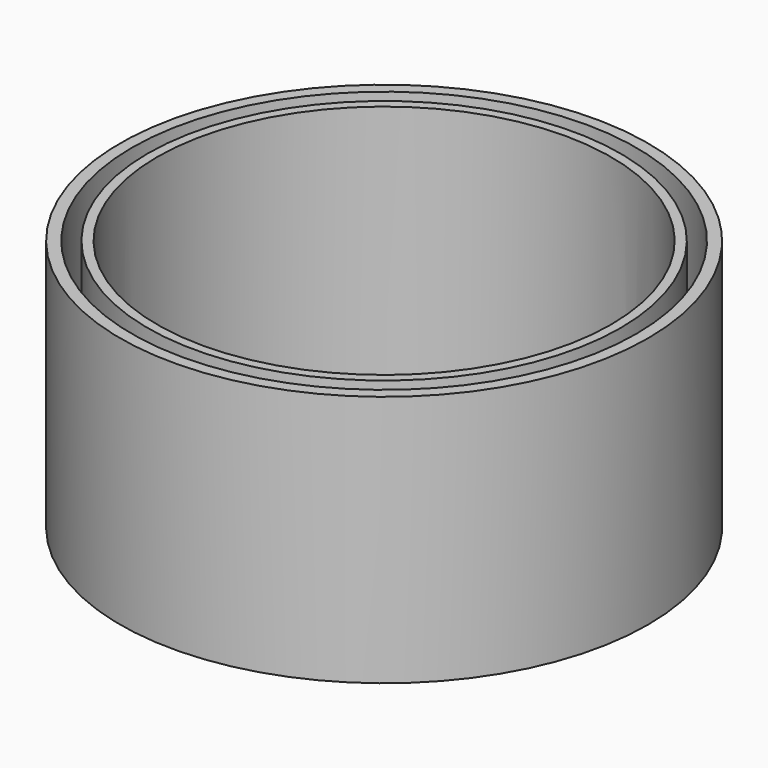
from build123d import *

# Parameters (mm, degrees)
F0_R      = 33.5
F0_R_2    = 32
F1_DEPTH  = 30
F0_R_3    = 30
F0_R_4    = 28.8
F2_R      = 33.5
F3_DEPTH  = 2
F5_DEPTH  = 12
F6_SIZE   = 11.9999
F6_2_SIZE = 11.9999
F6_3_SIZE = 11.9999
F8_R      = 6.5
F9_DEPTH  = 25


# Not quite as in the source:
# - a fillet or chamfer is up to 0.001 mm smaller than in the source, because OpenCascade refuses the exact size


with BuildPart() as f1:
    # F0 (on Top) → F1 (new body)
    with BuildSketch(Plane.XY):
        Circle(F0_R)
        Circle(F0_R_2, mode=Mode.SUBTRACT)
    extrude(amount=F1_DEPTH)


with BuildPart() as f1b:
    # F0 (on Top) → F1, piece 2 (new body)
    with BuildSketch(Plane.XY):
        Circle(F0_R_3)
        Circle(F0_R_4, mode=Mode.SUBTRACT)
    extrude(amount=F1_DEPTH)


with BuildPart() as f3:
    # F2 (on face) → F3 (new body)
    with BuildSketch(Plane(origin=(0, 0, 0), x_dir=(1, 0, 0), z_dir=(0, 0, -1))):
        Circle(F2_R)
    extrude(amount=F3_DEPTH)


with BuildPart() as f5:
    # F4 (on face) → F5 (new body)
    with BuildSketch(Plane.XY):
        with BuildLine():
            Line((9.993418715, 25.1754931604), (10.5667748746, 26.7914775395))
            ThreePointArc((10.5667748746, 26.7914775395), (10.0999818657, 26.9709170462), (9.630143492, 27.1422242332))
            Line((9.630143492, 27.1422242332), (9.993418715, 25.1754931604))
        make_face()
        with BuildLine():
            Line((8.1085420321, 25.8442531252), (9.630143492, 27.1422242332))
            ThreePointArc((9.630143492, 27.1422242332), (9.15740142, 27.3053474476), (8.6818981918, 27.4602375042))
            Line((8.6818981918, 27.4602375042), (8.1085420321, 25.8442531252))
        make_face()
        Polygon((9.993418715, 25.1754931604), (9.630143492, 27.1422242332), (5.6175837037, 15.832964136), (6.5600220451, 15.4985841536), align=None)
        Polygon((5.6175837037, 15.832964136), (9.630143492, 27.1422242332), (8.1085420321, 25.8442531252), (4.6751453622, 16.1673441184), align=None)
    extrude(amount=F5_DEPTH)

    # F6#2 (size 12 in the source; OpenCascade refuses exactly that, so slightly less here)
    f6_2_edges = [f5.edges().sort_by_distance(p)[0] for p in [
        (5.617584, 15.832964, 12),
    ]]
    chamfer(f6_2_edges, length=F6_2_SIZE)


with BuildPart() as f5b:
    # F4 (on face) → F5, piece 2 (new body)
    with BuildSketch(Plane.XY):
        with BuildLine():
            Line((-26.769701888, -3.9079218685), (-28.488352252, -4.2253740625))
            ThreePointArc((-28.488352252, -4.2253740625), (-28.4090912902, -4.7290096283), (-28.3209274471, -5.2311632104))
            Line((-28.3209274471, -5.2311632104), (-26.769701888, -3.9079218685))
        make_face()
        with BuildLine():
            ThreePointArc((-28.3209274471, -5.2311632104), (-28.2277588918, -5.7125850495), (-28.1264073572, -6.1923508604))
            Line((-28.1264073572, -6.1923508604), (-26.4727474785, -5.8869030696))
            Line((-26.4727474785, -5.8869030696), (-28.3209274471, -5.2311632104))
        make_face()
        Polygon((-16.7057304605, -2.0490040353), (-26.769701888, -3.9079218685), (-28.3209274471, -5.2311632104), (-16.5205565416, -3.0515147414), (-16.5240928491, -3.0323695717), align=None)
        Polygon((-28.3209274471, -5.2311632104), (-26.4727474785, -5.8869030696), (-16.3424552376, -4.0157351081), (-16.5205565416, -3.0515147414), align=None)
    extrude(amount=F5_DEPTH)

    # F6 (size 12 in the source; OpenCascade refuses exactly that, so slightly less here)
    f6_edges = [f5b.edges().sort_by_distance(p)[0] for p in [
        (-16.524093, -3.03237, 12),
    ]]
    chamfer(f6_edges, length=F6_SIZE)


with BuildPart() as f5c:
    # F4 (on face) → F5, piece 3 (new body)
    with BuildSketch(Plane.XY):
        with BuildLine():
            ThreePointArc((17.9187127168, -22.5468342472), (18.3075083925, -22.2322993966), (18.6907839551, -21.9110610228))
            Line((18.6907839551, -21.9110610228), (16.8059072723, -21.242301058))
            Line((16.8059072723, -21.242301058), (17.9187127168, -22.5468342472))
        make_face()
        with BuildLine():
            ThreePointArc((18.6907839551, -21.9110610228), (19.0684238388, -21.5832159862), (19.4403141767, -21.2488631392))
            Line((19.4403141767, -21.2488631392), (18.3275087322, -19.94432995))
            Line((18.3275087322, -19.94432995), (18.6907839551, -21.9110610228))
        make_face()
        Polygon((10.9029573072, -12.7814522633), (18.6907839551, -21.9110610228), (18.3275087322, -19.94432995), (11.6637580371, -12.1324667093), align=None)
        Polygon((16.8059072723, -21.242301058), (18.6907839551, -21.9110610228), (10.9029573072, -12.7814522633), (10.1421565772, -13.4304378173), align=None)
    extrude(amount=F5_DEPTH)

    # F6#3 (size 12 in the source; OpenCascade refuses exactly that, so slightly less here)
    f6_3_edges = [f5c.edges().sort_by_distance(p)[0] for p in [
        (10.902957, -12.781452, 12),
    ]]
    chamfer(f6_3_edges, length=F6_3_SIZE)


with BuildPart() as f5_1:
    add(f5.part)

    # F7: union F1b, F1, F3, F5b, F5c
    add(f1b.part)
    add(f1.part)
    add(f3.part)
    add(f5b.part)
    add(f5c.part)

    # F8 (on face) → F9 (cut)
    with BuildSketch(Plane.XY):
        Circle(F8_R)
    extrude(amount=-F9_DEPTH, mode=Mode.SUBTRACT)


solid = f5_1.part
